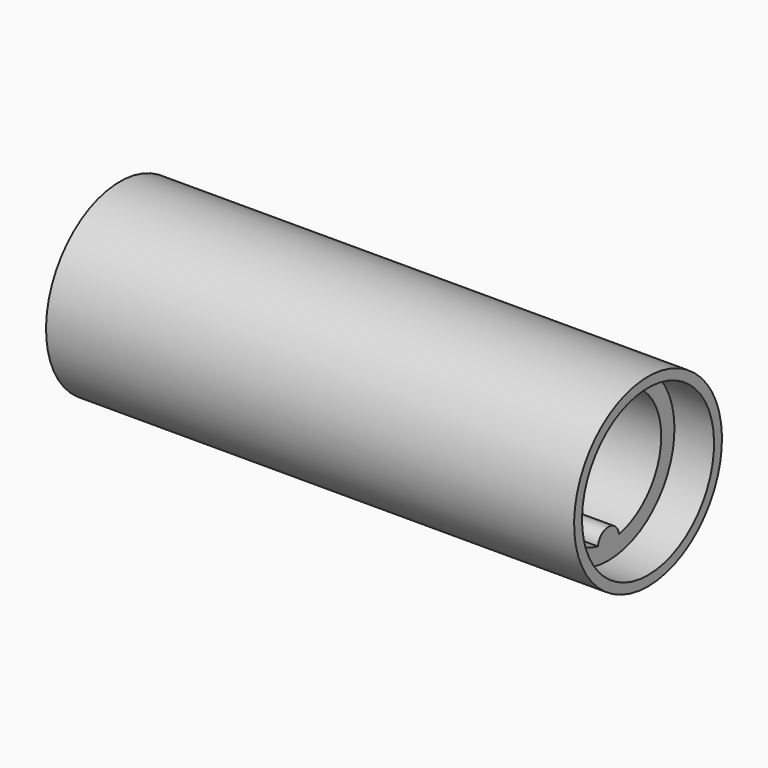
from build123d import *

# Parameters (mm, degrees)
F2_R     = 1
F3_DEPTH = 37
F5_R     = 1.5
F6_DEPTH = 27.001
F8_DEPTH = 3


# Not quite as in the source:
# - a fillet or chamfer that OpenCascade refuses, or shapes differently, is made with other operations: its cross-section is extruded or revolved along the edge and cut away or added


with BuildPart() as f1:
    # F0 (on Front) → F1 (revolve)
    with BuildSketch(Plane.XZ):
        Polygon((0, -7), (40, -7), (40, -6.25), (37, -6.25), (37, -5), (5, -5), (5, -4), (0, -4), align=None)
    revolve(axis=Axis((17.6803227514, 0, 0), (1, 0, 0)))

    # F2 (on face) → F3 (join, through all)
    with BuildSketch(Plane.YZ.offset(37)):
        with Locations((0, -5)):
            Circle(F2_R)
    extrude(amount=-F3_DEPTH)


with BuildPart() as f1b:
    # F0 (on Front) → F1, piece 2 (revolve)
    with BuildSketch(Plane.XZ):
        Polygon((0, -2), (0, -3.5), (22, -3.5), (22, -4.5), (27, -4.5), (27, -2), align=None)
    revolve(axis=Axis((17.6803227514, 0, 0), (1, 0, 0)))

    # F4: fillet of radius 2 on 1 edges, made by hand

    # F4_s1 → F4_t2 (revolve)
    with BuildSketch(Plane.XZ):
        with BuildLine():
            ThreePointArc((20.2679491924, -3.5), (21.2679491924, -3.7679491924), (22, -4.5))
            Line((22, -4.5), (22, -3.5))
            Line((22, -3.5), (20.2679491924, -3.5))
        make_face()
    revolve(axis=Axis((22, 0, 0), (1, 0, 0)))

    # F5 (on face) → F6 (cut, through all)
    with BuildSketch(Plane.YZ.offset(27)):
        with Locations((0, -5)):
            Circle(F5_R)
    extrude(amount=-F6_DEPTH, mode=Mode.SUBTRACT)

    # F7 (on face) → F8 (cut)
    with BuildSketch(Plane.YZ.offset(27)):
        Polygon((1.7320508076, 3), (-1.7320508076, 3), (-3.4641016151, 0), (-1.7320508076, -3), (1.7320508076, -3), (3.4641016151, 0), align=None)
    extrude(amount=-F8_DEPTH, mode=Mode.SUBTRACT)


solid = Compound([f1.part, f1b.part])
